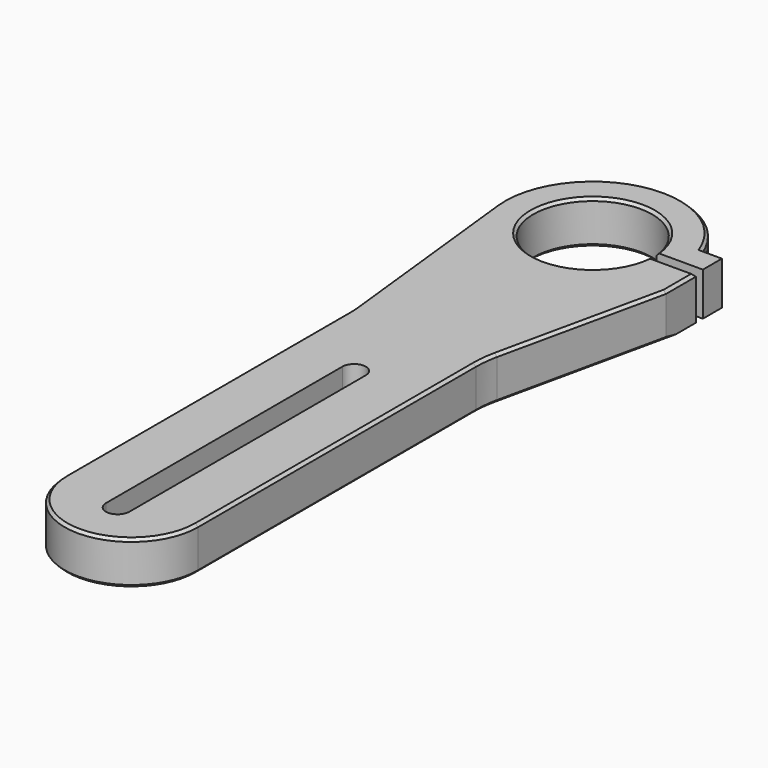
from build123d import *

# Parameters (mm, degrees)
F1_DEPTH      = 12
F3_DEPTH      = 2.5
F5_DEPTH      = 25
F6_R          = 30
F8_DEPTH      = 25
F8_DEPTH_BACK = 25
F9_R          = 4
F10_DEPTH     = 25
F11_R         = 1.8
F12_DEPTH     = 7.5
F13_SIZE      = 0.75
F14_SIZE      = 0.75
F15_SIZE      = 0.75
F16_W         = 5
F16_H         = 50.1374751329
F17_DEPTH     = 3
F18_R         = 2.49999


# Not quite as in the source:
# - a fillet or chamfer is up to 0.001 mm smaller than in the source, because OpenCascade refuses the exact size


with BuildPart() as f1:
    # F0 (on Top) → F1 (new body)
    with BuildSketch(Plane.XY):
        with BuildLine():
            Line((-3.74e-08, 99.6128183121), (0, 0))
            ThreePointArc((0, 0), (18.500000007, -18.499999993), (37, 1.39e-08))
            Line((37, 1.39e-08), (36.9999999626, 99.6128183121))
            Line((36.9999999626, 99.6128183121), (47.8017579937, 148.7838923931))
            Line((47.8017579937, 148.7838923931), (47.8017579937, 159.1853948904))
            Line((47.8017579937, 159.1853948904), (34.9798792017, 159.1853948904))
            ThreePointArc((34.9798792017, 159.1853948904), (2.004546746, 159.6126733438), (34.9234827971, 161.5872028336))
            Line((34.9234827971, 161.5872028336), (47.8017579834, 161.5872028336))
            Line((47.8017579834, 161.5872028336), (47.8017578313, 168.1936387276))
            Line((47.8017578313, 168.1936387276), (42.1191508, 168.1936387276))
            ThreePointArc((42.1191508, 168.1936387276), (13.0001519828, 184.387531079), (-6.3497242683, 157.2629936512))
            Line((-6.3497242683, 157.2629936512), (-3.74e-08, 99.6128183121))
        make_face()
    extrude(amount=F1_DEPTH)

    # F2 (on face) → F3 (join)
    with BuildSketch(Plane(origin=(0, 0, 0), x_dir=(1, 0, 0), z_dir=(0, 0, -1))):
        with BuildLine():
            ThreePointArc((29.3, -7e-09), (18.5, 10.799999993), (7.7, -7e-09))
            Line((7.7, -7e-09), (7.7, -72.500000007))
            ThreePointArc((7.7, -72.500000007), (18.5, -83.300000007), (29.3, -72.500000007))
            Line((29.3, -72.500000007), (29.3, -7e-09))
        make_face()
    extrude(amount=F3_DEPTH)

    # F4 (on face) → F5 (cut)
    with BuildSketch(Plane(origin=(0, 0, -2.5), x_dir=(1, 0, 0), z_dir=(0, 0, -1))):
        with BuildLine():
            ThreePointArc((21.75, 4.749999993), (18.5, 7.999999993), (15.25, 4.749999993))
            Line((15.25, 4.749999993), (15.25, -77.250000007))
            ThreePointArc((15.25, -77.250000007), (18.5, -80.500000007), (21.75, -77.250000007))
            Line((21.75, -77.250000007), (21.75, 4.749999993))
        make_face()
    extrude(amount=-F5_DEPTH, mode=Mode.SUBTRACT)

    # F6
    f6_edges = [f1.edges().sort_by_distance(p)[0] for p in [
        (0, 99.612818, 6),
        (37, 99.612818, 6),
    ]]
    fillet(f6_edges, radius=F6_R)

    # F7 (on face) → F8 (cut, two sides)
    with BuildSketch(Plane(origin=(0, 168.1936387276, 0), x_dir=(-1, 0, 0), z_dir=(0, 1, 0))) as f8_sk:
        with BuildLine():
            ThreePointArc((-42.1191508, 4.5), (-41.0584906283, 4.9393398282), (-40.6191508, 6))
            ThreePointArc((-40.6191508, 6), (-41.0584906283, 7.0606601718), (-42.1191508, 7.5))
            Line((-42.1191508, 7.5), (-42.1191508, 4.5))
        make_face()
        with BuildLine():
            Line((-42.1191508, 4.5), (-42.1191508, 7.5))
            ThreePointArc((-42.1191508, 7.5), (-43.6191508, 6), (-42.1191508, 4.5))
        make_face()
    extrude(amount=-F8_DEPTH, mode=Mode.SUBTRACT)
    extrude(f8_sk.sketch, amount=F8_DEPTH_BACK, mode=Mode.SUBTRACT)

    # F9 (on face) → F10 (cut)
    with BuildSketch(Plane(origin=(0, 168.1936387276, 0), x_dir=(-1, 0, 0), z_dir=(0, 1, 0))):
        with Locations((-42.1191508, 6)):
            Circle(F9_R)
    extrude(amount=F10_DEPTH, mode=Mode.SUBTRACT)

    # F11 (on face) → F12 (cut)
    with BuildSketch(Plane(origin=(0, 168.1936387276, 0), x_dir=(-1, 0, 0), z_dir=(0, 1, 0))):
        with Locations((-42.1191508, 6)):
            Circle(F11_R)
    extrude(amount=-F12_DEPTH, mode=Mode.SUBTRACT)

    # F13
    f13_edges = [f1.edges().sort_by_distance(p)[0] for p in [
        (37, 48.178243, 12),
        (41.390819, 159.185395, 12),
        (2.004547, 159.612673, 12),
        (47.801758, 153.984644, 12),
    ]]
    chamfer(f13_edges, length=F13_SIZE)

    # F14
    f14_edges = [f1.edges().sort_by_distance(p)[0] for p in [
        (2.004547, 159.612673, 0),
    ]]
    chamfer(f14_edges, length=F14_SIZE)

    # F15
    f15_edges = [f1.edges().sort_by_distance(p)[0] for p in [
        (42.75022, 125.788603, 0),
        (13.000152, 184.387531, 0),
        (-3.265028, 129.256533, 0),
        (37.175182, 99.593803, 0),
        (-0.045117, 99.610341, 0),
        (37, 48.178243, 0),
        (0, 48.982832, 0),
        (18.5, -18.5, 0),
    ]]
    chamfer(f15_edges, length=F15_SIZE)

    # F16 (on face) → F17 (cut)
    with BuildSketch(Plane(origin=(0, 0, 0), x_dir=(1, 0, 0), z_dir=(0, 0, -1))):
        with Locations((25, -111.8474081159)):
            Rectangle(F16_W, F16_H)
        with Locations((12, -111.8474081159)):
            Rectangle(F16_W, F16_H)
    extrude(amount=-F17_DEPTH, mode=Mode.SUBTRACT)

    # F18 (radius 2.5 in the source; OpenCascade refuses exactly that, so slightly less here)
    f18_edges = [f1.edges().sort_by_distance(p)[0] for p in [
        (22.5, 136.916146, 1.5),
        (27.5, 136.916146, 1.5),
        (14.5, 136.916146, 1.5),
        (9.5, 136.916146, 1.5),
        (9.5, 86.778671, 1.5),
        (14.5, 86.778671, 1.5),
        (27.5, 86.778671, 1.5),
        (22.5, 86.778671, 1.5),
    ]]
    fillet(f18_edges, radius=F18_R)


solid = f1.part
